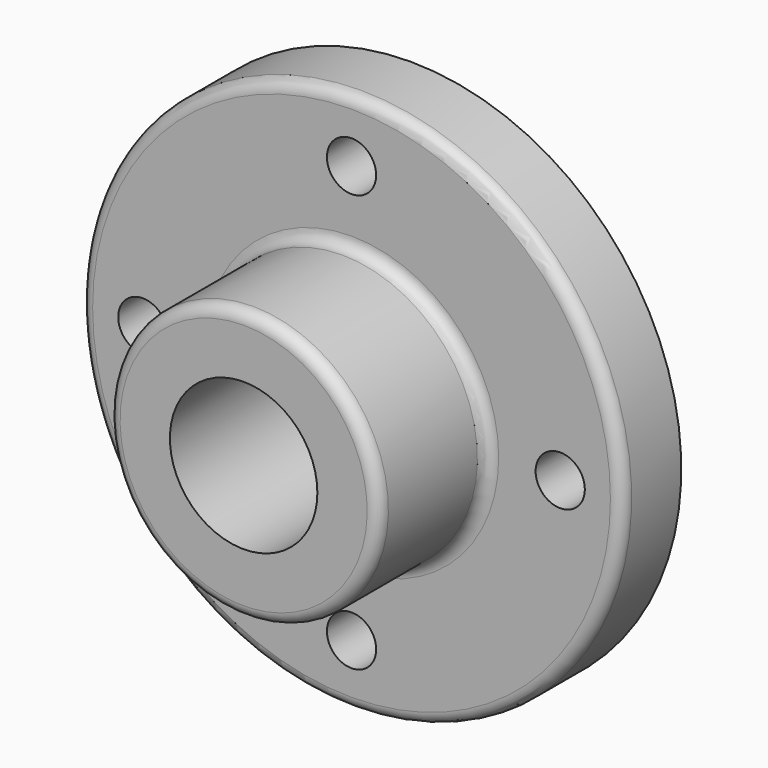
from build123d import *

# Parameters (mm, degrees)
F2_R     = 19.0246
F3_DEPTH = 53.849
F4_R     = 6.35
F5_DEPTH = 19.051
F6_R     = 3.048


# Not quite as in the source:
# - a feature names something its author has since deleted; it is built from what else it names


with BuildPart() as f1:
    # F0 (on Right) → F1 (revolve)
    with BuildSketch(Plane.YZ):
        Polygon((0, 34.925), (0, 0), (53.848, 0), (53.848, 69.85), (34.798, 69.85), (34.798, 34.925), align=None)
    revolve(axis=Axis((0, 26.924, 0), (0, 1, 0)))

    # F2 (on face) → F3 (cut, through all)
    with BuildSketch(Plane.XZ):
        Circle(F2_R)
    extrude(amount=-F3_DEPTH, mode=Mode.SUBTRACT)

    # F4 (on face) → F5 (cut, through all)
    with BuildSketch(Plane.XZ.offset(-34.798)):
        with Locations((0, 53.848)):
            Circle(F4_R)
        with Locations((-53.848, 0)):
            Circle(F4_R)
        with Locations((53.848, 0)):
            Circle(F4_R)
        with Locations((0, -53.848)):
            Circle(F4_R)
    extrude(amount=-F5_DEPTH, mode=Mode.SUBTRACT)

    # F6
    f6_edges = [f1.edges().sort_by_distance(p)[0] for p in [
        (0, 34.798, -34.925),
        (0, 0, -34.925),
        (0, 34.798, -69.85),
    ]]
    fillet(f6_edges, radius=F6_R)


solid = f1.part
